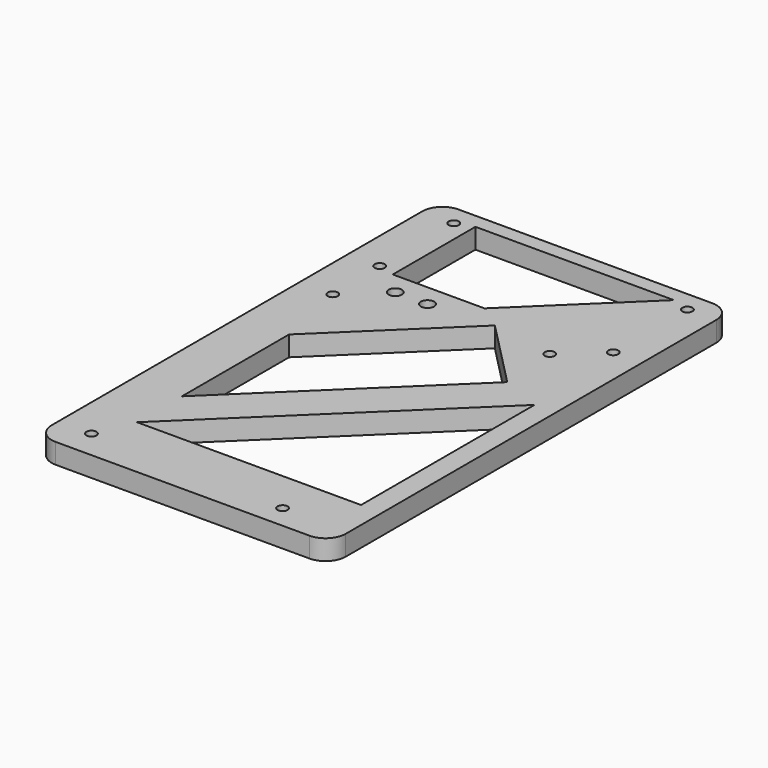
from build123d import *

# Parameters (mm, degrees)
F0_W     = 73
F0_H     = 125
F1_DEPTH = 5
F2_D     = 2.5
F3_D     = 3.3
F4_R     = 5
F7_DEPTH = 25
F8_D     = 2.5


# Not quite as in the source:
# - a feature names something its author has since deleted; it is built from what else it names


with BuildPart() as f1:
    # F0 (on Top) → F1 (new body)
    with BuildSketch(Plane.XY):
        with Locations((-1.7126457989, 19.3158909678)):
            Rectangle(F0_W, F0_H)
    extrude(amount=F1_DEPTH)

    # F2 (through all)
    with Locations(Plane(origin=(0, 0, 0), x_dir=(1, 0, 0), z_dir=(0, 0, -1))):
        with Locations((-30.3091388196, -76.7177641392), (27.6908611804, -76.7177641392), (27.6908611804, -53.7177641392), (-30.3091388196, -53.7177641392)):
            Hole(F2_D / 2)

    # F3 (through all)
    with Locations(Plane(origin=(0, 0, 0), x_dir=(1, 0, 0), z_dir=(0, 0, -1))):
        with Locations((-21.0855398327, -47.0293052495), (-13.0855398327, -47.0293052495)):
            Hole(F3_D / 2)

    # F4
    f4_edges = [f1.edges().sort_by_distance(p)[0] for p in [
        (-38.212646, 81.815891, 2.5),
        (34.787354, 81.815891, 2.5),
        (34.787354, -43.184109, 2.5),
        (-38.212646, -43.184109, 2.5),
    ]]
    fillet(f4_edges, radius=F4_R)

    # F5 (on face) → F7 (cut)
    with BuildSketch(Plane.XY.offset(5)):
        Polygon((19.4577450805, 31.105422746), (2.7185706181, 48.1802586667), (-26.0799791984, 20.3202102417), (-26.0799791984, -12.9482956412), align=None)
        Polygon((29.5474557331, 26.9350063375), (-26.0799791984, -26.8796142191), (29.5474557331, -26.8796142191), align=None)
        Polygon((-3.3391041424, 52.5376833975), (23.1605084746, 78.173713526), (-26.1079283048, 78.173713526), (-26.1079283048, 52.5376833975), align=None)
    extrude(amount=-F7_DEPTH, mode=Mode.SUBTRACT)

    # F8 (through all)
    with Locations(Plane.XY.offset(5)):
        with Locations((-29.995566234, 38.7779349625), (18.504433766, 45.4779349625), (18.504433766, -37.4220650375), (-29.995566234, -36.1220650375)):
            Hole(F8_D / 2)


solid = f1.part
